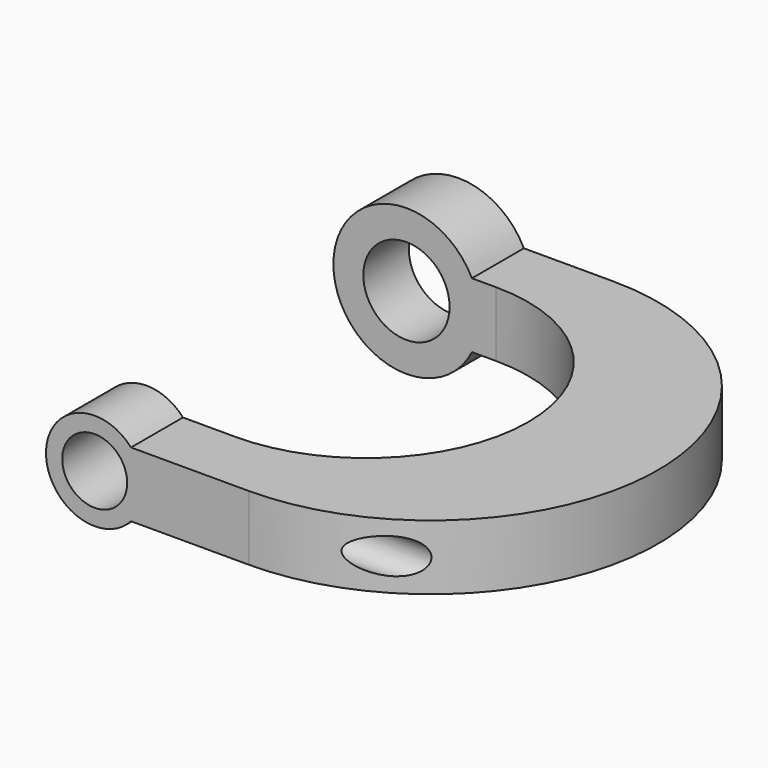
from build123d import *

# Parameters (mm, degrees)
F1_DEPTH       = 44.45
F3_DEPTH       = 12.7
F5_D           = 8.4328
F5_DEPTH       = 6.35
F5_CBORE_D     = 12.7
F5_CBORE_DEPTH = 0.79375
F5_TIP         = 2.5334687141
F6_R           = 3.175
F7_DEPTH       = 25.4
F8_R           = 1.7272
F9_DEPTH       = 38.1


# Not quite as in the source:
# - a feature names something its author has since deleted; it is built from what else it names


with BuildPart() as f1:
    # F0 (on Front) → F1 (new body)
    with BuildSketch(Plane.XZ):
        with BuildLine():
            Line((-30.9068329123, 0), (0, 0))
            Line((0, 0), (0, 6.35))
            Line((0, 6.35), (-30.9068329123, 6.35))
            ThreePointArc((-30.9068329123, 6.35), (-30.3510720769, 4.8055410516), (-30.1625, 3.175))
            ThreePointArc((-30.1625, 3.175), (-30.3510720769, 1.5444589484), (-30.9068329123, 0))
        make_face()
        with BuildLine():
            ThreePointArc((-43.7056670877, 0), (-37.30625, -3.96875), (-30.9068329123, 0))
            Line((-30.9068329123, 0), (-43.7056670877, 0))
        make_face()
        with BuildLine():
            Line((-43.7056670877, 0), (-30.9068329123, 0))
            ThreePointArc((-30.9068329123, 0), (-30.3510720769, 1.5444589484), (-30.1625, 3.175))
            ThreePointArc((-30.1625, 3.175), (-30.3510720769, 4.8055410516), (-30.9068329123, 6.35))
            Line((-30.9068329123, 6.35), (-43.7056670877, 6.35))
            ThreePointArc((-43.7056670877, 6.35), (-44.2614279231, 4.8055410516), (-44.45, 3.175))
            ThreePointArc((-44.45, 3.175), (-44.2614279231, 1.5444589484), (-43.7056670877, 0))
        make_face()
        with BuildLine():
            Line((-43.7056670877, 6.35), (-30.9068329123, 6.35))
            ThreePointArc((-30.9068329123, 6.35), (-37.30625, 10.31875), (-43.7056670877, 6.35))
        make_face()
    extrude(amount=F1_DEPTH)

    # F2 (on face) → F3 (intersect, symmetric)
    with BuildSketch(Plane.XY.offset(6.35)):
        with BuildLine():
            Line((-22.225, 0), (-44.45, 0))
            Line((-44.45, 0), (-44.45, -6.35))
            Line((-44.45, -6.35), (-28.575, -6.35))
            ThreePointArc((-28.575, -6.35), (-12.7, -22.225), (-28.575, -38.1))
            Line((-28.575, -38.1), (-44.45, -38.1))
            Line((-44.45, -38.1), (-44.45, -44.45))
            Line((-44.45, -44.45), (-22.225, -44.45))
            ThreePointArc((-22.225, -44.45), (0, -22.225), (-22.225, 0))
        make_face()
    extrude(amount=F3_DEPTH, both=True, mode=Mode.INTERSECT)

    # F5
    with Locations(Plane(origin=(0, 0, 0), x_dir=(-1, 0, 0), z_dir=(0, 1, 0))):
        with Locations((37.30625, 3.175)):
            CounterBoreHole(F5_D / 2, F5_CBORE_D / 2, F5_CBORE_DEPTH, depth=F5_DEPTH)
            with Locations((0, 0, -(F5_DEPTH + F5_TIP / 2))):  # 118° drill point
                Cone(0, F5_D / 2, F5_TIP, mode=Mode.SUBTRACT)

    # F6 (on face) → F7 (cut)
    with BuildSketch(Plane.XZ.offset(44.45)):
        with BuildLine():
            ThreePointArc((-33.7564920857, 0), (-42.06875, 3.175), (-33.7564920857, 6.35))
            Line((-33.7564920857, 6.35), (-30.9068329123, 6.35))
            ThreePointArc((-30.9068329123, 6.35), (-44.45, 3.175), (-30.9068329123, 0))
            Line((-30.9068329123, 0), (-33.7564920857, 0))
        make_face()
        with Locations((-37.30625, 3.175)):
            Circle(F6_R)
    extrude(amount=-F7_DEPTH, mode=Mode.SUBTRACT)

    # F8 (on Right) → F9 (cut)
    with BuildSketch(Plane.YZ):
        with Locations((-41.275, 3.175)):
            Circle(F8_R)
    extrude(amount=-F9_DEPTH, mode=Mode.SUBTRACT)


solid = f1.part
